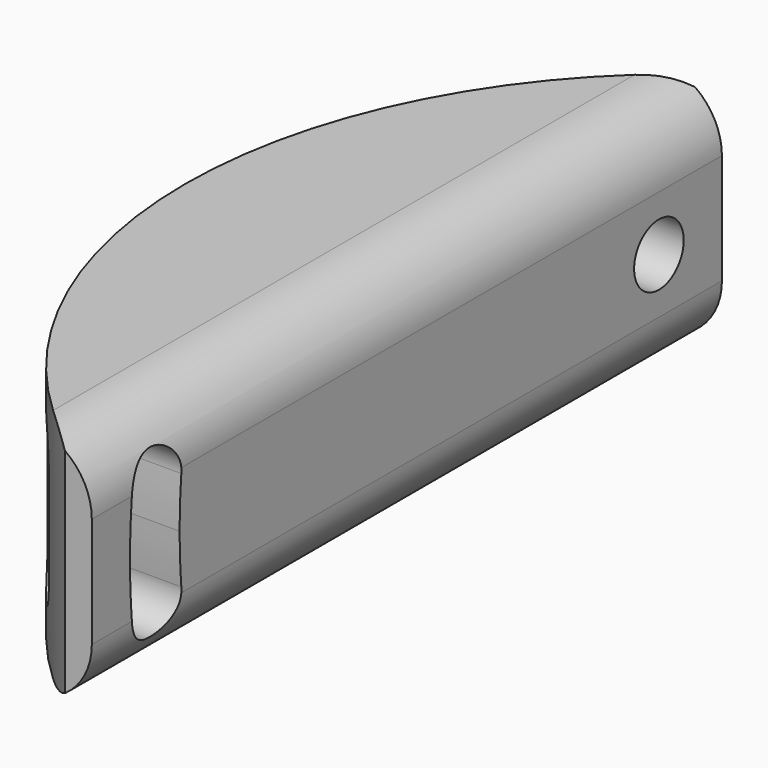
from build123d import *

# Parameters (mm, degrees)
F1_DEPTH    = 19.05
F3_DEPTH    = 25.4
F4_D        = 5
F4_DEPTH    = 15.6972
F4_TIP      = 1.5021515476
F5_T1_DEPTH = 88.9


# Not quite as in the source:
# - a fillet or chamfer that OpenCascade refuses, or shapes differently, is made with other operations: its cross-section is extruded or revolved along the edge and cut away or added


with BuildPart() as f1:
    # F0 (on Top) → F1 (new body)
    with BuildSketch(Plane.XY):
        with BuildLine():
            Line((-22.0673531294, 31.75), (-24.2402065279, 31.75))
            ThreePointArc((-24.2402065279, 31.75), (-39.9455894, 0), (-24.2402065279, -31.75))
            Line((-24.2402065279, -31.75), (-22.0673531294, -31.75))
            Line((-22.0673531294, -31.75), (-22.0673531294, 31.75))
        make_face()
    extrude(amount=F1_DEPTH)

    # F2 (on face) → F3 (cut)
    with BuildSketch(Plane.YZ.offset(-22.0673531294)):
        with BuildLine():
            ThreePointArc((-27.7153407028, 13.9654662391), (-27.8542875294, 11.747165191), (-27.90063, 9.525))
            Line((-27.90063, 9.525), (-22.89937, 9.525))
            ThreePointArc((-22.89937, 9.525), (-22.8573758972, 11.538656851), (-22.7314666127, 13.5488121361))
            ThreePointArc((-22.7314666127, 13.5488121361), (-25.0150766063, 16.2490762326), (-27.7153407028, 13.9654662391))
        make_face()
        with BuildLine():
            Line((-22.89937, 9.525), (-27.90063, 9.525))
            ThreePointArc((-27.90063, 9.525), (-27.8542875294, 7.302834809), (-27.7153407028, 5.0845337609))
            ThreePointArc((-27.7153407028, 5.0845337609), (-25.0150766063, 2.8009237674), (-22.7314666127, 5.5011878639))
            ThreePointArc((-22.7314666127, 5.5011878639), (-22.8573758972, 7.511343149), (-22.89937, 9.525))
        make_face()
    extrude(amount=-F3_DEPTH, mode=Mode.SUBTRACT)

    # F4
    with Locations(Plane.YZ.offset(-22.0673531294)):
        with Locations((25.4, 9.525)):
            Hole(F4_D / 2, depth=F4_DEPTH)
            with Locations((0, 0, -(F4_DEPTH + F4_TIP / 2))):  # 118° drill point
                Cone(0, F4_D / 2, F4_TIP, mode=Mode.SUBTRACT)

    # F5: fillet of radius 5.08 on 2 edges, made by hand

    # F5_s2 → F5_t1 (cut)
    with BuildSketch(Plane.XZ.offset(-44.45)):
        with BuildLine():
            ThreePointArc((-22.0673531294, 13.97), (-23.555250681, 17.5621024484), (-27.1473531294, 19.05))
            Line((-27.1473531294, 19.05), (-22.0673531294, 19.05))
            Line((-22.0673531294, 19.05), (-22.0673531294, 13.97))
        make_face()
        with BuildLine():
            ThreePointArc((-22.0673531294, 5.08), (-23.555250681, 1.4878975516), (-27.1473531294, 0))
            Line((-27.1473531294, 0), (-22.0673531294, 0))
            Line((-22.0673531294, 0), (-22.0673531294, 5.08))
        make_face()
    extrude(amount=F5_T1_DEPTH, mode=Mode.SUBTRACT)


solid = f1.part
